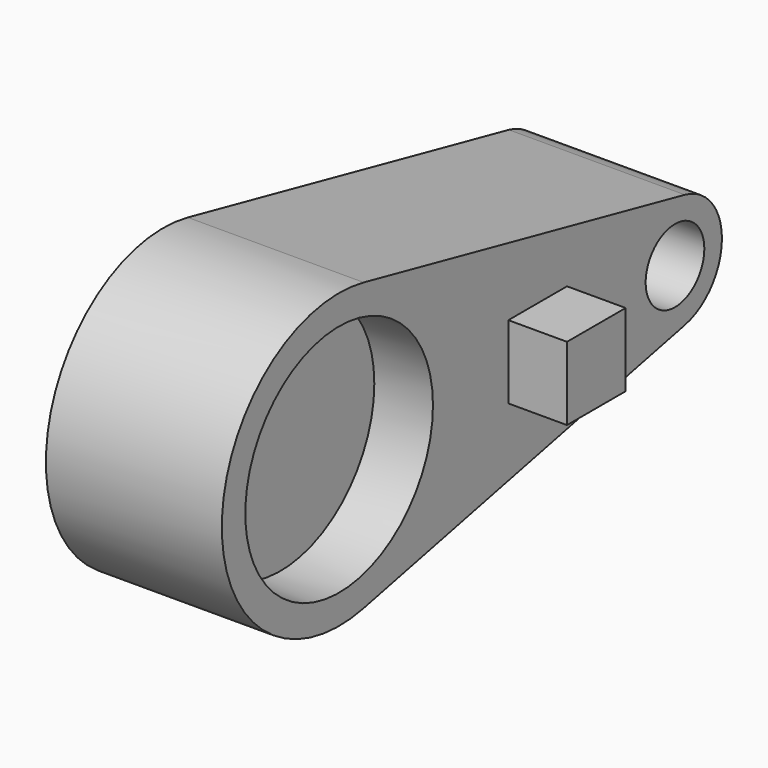
from build123d import *

# Parameters (mm, degrees)
F1_DEPTH = 76.2
F2_R     = 50.8
F3_DEPTH = 25.4
F4_W     = 31.75
F4_H     = 31.75
F5_DEPTH = 25.4
F6_R     = 15.875
F7_DEPTH = 76.2


with BuildPart() as f1:
    # F0 (on Right) → F1 (new body)
    with BuildSketch(Plane.YZ):
        with BuildLine():
            ThreePointArc((13.3050971344, -62.0904532939), (49.3817965856, -39.9210241099), (63.5, 0))
            ThreePointArc((63.5, 0), (49.3817965856, 39.9210241099), (13.3050971344, 62.0904532939))
            ThreePointArc((13.3050971344, 62.0904532939), (-63.5, 0), (13.3050971344, -62.0904532939))
        make_face()
        with BuildLine():
            ThreePointArc((13.3050971344, 62.0904532939), (49.3817965856, 39.9210241099), (63.5, 0))
            ThreePointArc((63.5, 0), (49.3817965856, -39.9210241099), (13.3050971344, -62.0904532939))
            Line((13.3050971344, -62.0904532939), (187.1583663574, -24.8361813176))
            ThreePointArc((187.1583663574, -24.8361813176), (156.4363275036, 0), (187.1583663574, 24.8361813176))
            Line((187.1583663574, 24.8361813176), (13.3050971344, 62.0904532939))
        make_face()
        with BuildLine():
            ThreePointArc((207.2363275036, 0), (201.5890461378, 15.968409644), (187.1583663574, 24.8361813176))
            ThreePointArc((187.1583663574, 24.8361813176), (156.4363275036, 0), (187.1583663574, -24.8361813176))
            ThreePointArc((187.1583663574, -24.8361813176), (201.5890461378, -15.968409644), (207.2363275036, 0))
        make_face()
    extrude(amount=F1_DEPTH)

    # F2 (on face) → F3 (cut)
    with BuildSketch(Plane.YZ.offset(76.2)):
        Circle(F2_R)
    extrude(amount=-F3_DEPTH, mode=Mode.SUBTRACT)

    # F4 (on face) → F5 (join)
    with BuildSketch(Plane.YZ.offset(76.2)):
        with Locations((107.4921913939, 0)):
            Rectangle(F4_W, F4_H)
    extrude(amount=F5_DEPTH)

    # F6 (on face) → F7 (cut, through all)
    with BuildSketch(Plane.YZ.offset(76.2)):
        with Locations((181.8363275036, 0)):
            Circle(F6_R)
    extrude(amount=-F7_DEPTH, mode=Mode.SUBTRACT)


solid = f1.part
